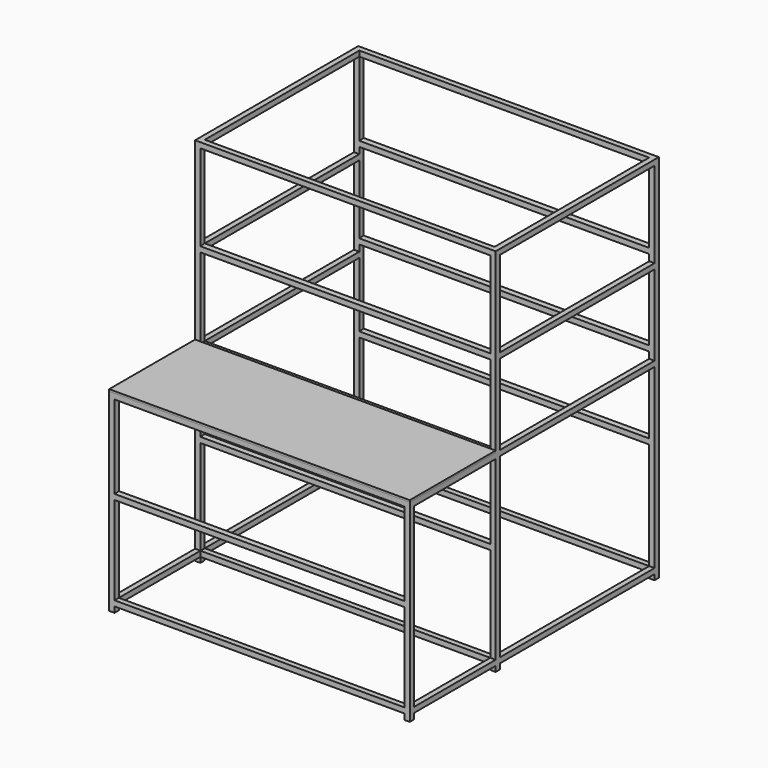
from build123d import *

# Parameters (mm, degrees)
F0_W      = 25.4
F0_H      = 914.4
F0_H_2    = 25.4
F0_W_2    = 1371.6
F1_DEPTH  = 25.4
F2_DEPTH  = 1727.2
F4_DEPTH  = 1422.4
F6_W      = 1422.4
F6_H      = 965.2
F6_W_2    = 1371.6
F6_H_2    = 914.4
F7_DEPTH  = 25.4
F8_W      = 25.4
F8_H      = 25.4474646512
F9_DEPTH  = 914.4
F10_W     = 25.4
F10_H     = 25.4474646512
F10_H_2   = 25.4
F11_DEPTH = 508
F12_W     = 25.4
F12_H     = 25.4
F13_DEPTH = 914.4
F14_W     = 25.4
F14_H     = 25.4
F15_DEPTH = 914.4
F16_W     = 25.4
F16_H     = 25.4474646512
F16_H_2   = 25.4
F17_DEPTH = 1371.6
F18_W     = 1422.4
F18_H     = 508
F19_DEPTH = 9.525
F21_DEPTH = 1422.4


# Not quite as in the source:
# - a feature names something its author has since deleted; it is built from what else it names


with BuildPart() as f1:
    # F0 (on Top) → F1 (new body)
    with BuildSketch(Plane.XY):
        with Locations((698.5, 0)):
            Rectangle(F0_W, F0_H)
        with Locations((698.5, 469.9)):
            Rectangle(F0_W, F0_H_2)
        with Locations((0, 469.9)):
            Rectangle(F0_W_2, F0_H_2)
        with Locations((-698.5, 0)):
            Rectangle(F0_W, F0_H)
        with Locations((-698.5, 469.9)):
            Rectangle(F0_W, F0_H_2)
        with Locations((0, -469.9)):
            Rectangle(F0_W_2, F0_H_2)
        with Locations((698.5, -469.9)):
            Rectangle(F0_W, F0_H_2)
        with Locations((-698.5, -469.9)):
            Rectangle(F0_W, F0_H_2)
    extrude(amount=F1_DEPTH)

    # F0 (on Top) → F2 (join)
    with BuildSketch(Plane.XY):
        with Locations((-698.5, -469.9)):
            Rectangle(F0_W, F0_H_2)
        with Locations((-698.5, 469.9)):
            Rectangle(F0_W, F0_H_2)
        with Locations((698.5, 469.9)):
            Rectangle(F0_W, F0_H_2)
        with Locations((698.5, -469.9)):
            Rectangle(F0_W, F0_H_2)
    extrude(amount=-F2_DEPTH)

    # F3 (on face) → F4 (join)
    with BuildSketch(Plane.YZ.offset(711.2)):
        Polygon((-457.2, -431.8474646512), (-457.2, -406.4), (-482.6, -407.9535305518), (-482.6, -433.400995203), align=None)
        Polygon((482.6, -348.9193695826), (457.2, -350.4729001344), (457.2, -375.9203647856), (482.6, -374.3668342338), align=None)
        Polygon((482.6, -755.3193695826), (457.2, -756.8729001344), (457.2, -782.3203647856), (482.6, -780.7668342338), align=None)
        Polygon((-457.2, -838.2474646512), (-457.2, -812.8), (-482.6, -814.3535305518), (-482.6, -839.800995203), align=None)
    extrude(amount=-F4_DEPTH)

    # F6 (on offset) → F7 (join)
    with BuildSketch(Plane.XY.offset(-1676.4)):
        Rectangle(F6_W, F6_H)
        Rectangle(F6_W_2, F6_H_2, mode=Mode.SUBTRACT)
    extrude(amount=-F7_DEPTH)

    # F8 (on face) → F9 (join)
    with BuildSketch(Plane(origin=(0, -457.2, 0), x_dir=(-1, 0, 0), z_dir=(0, 1, 0))):
        with Locations((-698.5, -825.5237323256)):
            Rectangle(F8_W, F8_H)
        with Locations((698.5, -825.5237323256)):
            Rectangle(F8_W, F8_H)
        with Locations((-698.5, -419.1237323256)):
            Rectangle(F8_W, F8_H)
        with Locations((698.5, -419.1237323256)):
            Rectangle(F8_W, F8_H)
    extrude(amount=F9_DEPTH)

    # F10 (on face) → F11 (join)
    with BuildSketch(Plane.XZ.offset(482.6)):
        with Locations((-698.5, -827.0772628774)):
            Rectangle(F10_W, F10_H)
        with Locations((698.5, -827.0772628774)):
            Rectangle(F10_W, F10_H)
        with Locations((-698.5, -1689.1)):
            Rectangle(F10_W, F10_H_2)
        with Locations((698.5, -1689.1)):
            Rectangle(F10_W, F10_H_2)
    extrude(amount=F11_DEPTH)

    # F12 (on face) → F13 (join)
    with BuildSketch(Plane.XY.offset(-814.3535305518)):
        with Locations((-698.5, -977.9)):
            Rectangle(F12_W, F12_H)
    extrude(amount=-F13_DEPTH)

    # F14 (on face) → F15 (join)
    with BuildSketch(Plane.XY.offset(-814.3535305518)):
        with Locations((698.5, -977.9)):
            Rectangle(F14_W, F14_H)
    extrude(amount=-F15_DEPTH)

    # F16 (on face) → F17 (join)
    with BuildSketch(Plane.YZ.offset(-685.8)):
        with Locations((-977.9, -827.0772628774)):
            Rectangle(F16_W, F16_H)
        with Locations((-977.9, -1689.1)):
            Rectangle(F16_W, F16_H_2)
    extrude(amount=F17_DEPTH)

    # F20 (on face) → F21 (join)
    with BuildSketch(Plane.YZ.offset(711.2)):
        Polygon((482.6, -1168.4474646512), (482.6, -1143.0474646512), (457.2, -1144.600995203), (457.2, -1170.000995203), align=None)
        Polygon((-457.2, -1225.9280950687), (-457.2, -1200.5280950687), (-482.6, -1202.0816256205), (-482.6, -1227.4816256205), align=None)
        Polygon((-965.2, -1256.9987061051), (-965.2, -1231.5987061051), (-990.6, -1233.1522366569), (-990.6, -1258.5522366569), align=None)
    extrude(amount=-F21_DEPTH)


with BuildPart() as f19:
    # F18 (on face) → F19 (new body)
    with BuildSketch(Plane.XY.offset(-814.3535305518)):
        with Locations((0, -736.6)):
            Rectangle(F18_W, F18_H)
    extrude(amount=F19_DEPTH)


solid = Compound([f1.part, f19.part])
